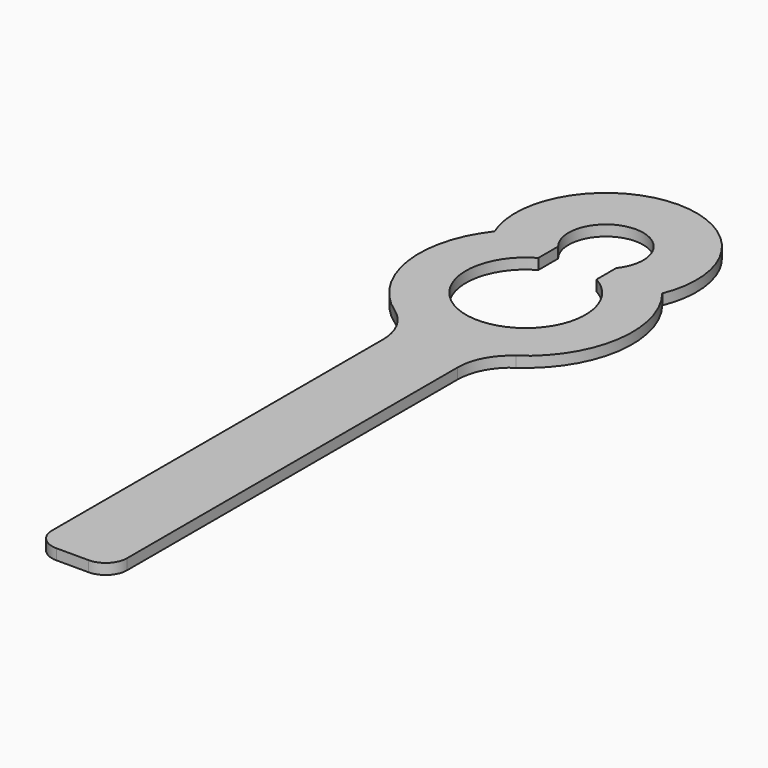
from build123d import *

# Parameters (mm, degrees)
F2_DEPTH = 1


# Not quite as in the source:
# - ends of sketch curves that miss each other by under 0.0002 mm in the source are joined


with BuildPart() as f2:
    # F1 (on Top) → F2 (new body)
    with BuildSketch(Plane.XY):
        with BuildLine():
            Line((-1.534358, -35.5), (1.499849, -35.5))
            ThreePointArc((1.499849, -35.5), (2.9140625624, -34.9142135624), (3.499849, -33.5))
            Line((3.499849, -33.5), (3.499849, 5.24069))
            ThreePointArc((3.499849, 5.24069), (4.0745571603, 7.568090295), (5.6665658533, 9.3604602133))
            ThreePointArc((5.6665658533, 9.3604602133), (9.8857158615, 16.0924782241), (7.8648732423, 23.7760641903))
            ThreePointArc((7.8648732423, 23.7760641903), (1.896e-07, 35.5), (-7.8648736534, 23.7760641421))
            ThreePointArc((-7.8648736534, 23.7760641421), (-9.8878127884, 16.1062937833), (-5.6895721633, 9.376328764))
            ThreePointArc((-5.6895721633, 9.376328764), (-4.1058182159, 7.585707204), (-3.534358, 5.264493))
            Line((-3.534358, 5.264493), (-3.534358, -33.5))
            ThreePointArc((-3.534358, -33.5), (-2.9485715624, -34.9142135624), (-1.534358, -35.5))
        make_face()
        with BuildLine():
            Line((-2.729304, 22.489878), (-2.729304, 24.808904))
            ThreePointArc((-2.729304, 24.808904), (3.13e-07, 30.5), (2.7293033847, 24.8089036912))
            Line((2.7293033847, 24.8089036912), (2.729303, 22.489878))
            ThreePointArc((2.729303, 22.489878), (4.366e-07, 12), (-2.729304, 22.489878))
        make_face(mode=Mode.SUBTRACT)
    extrude(amount=F2_DEPTH)


solid = f2.part
